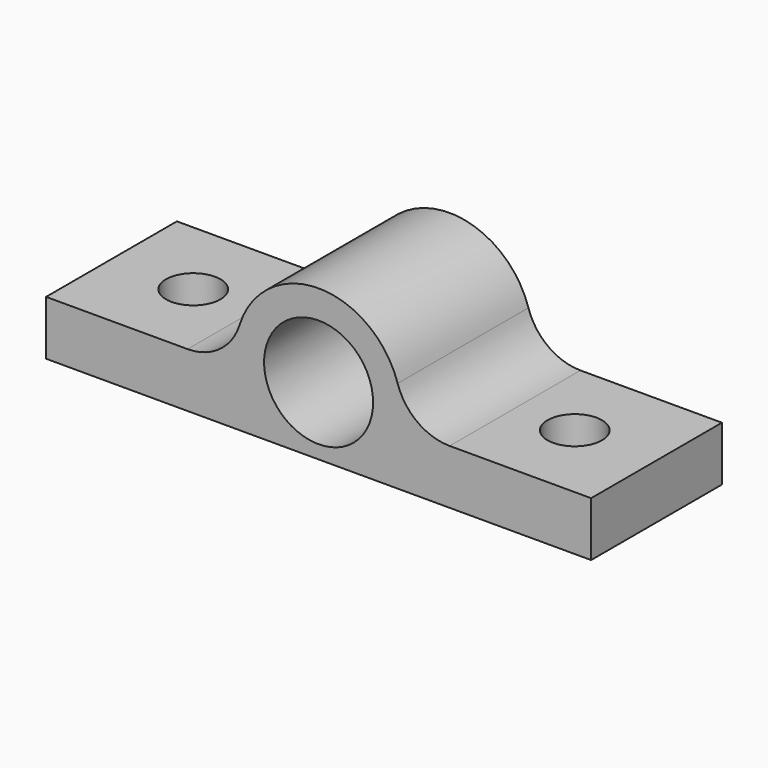
from build123d import *

# Parameters (mm, degrees)
F0_R     = 12.7
F1_DEPTH = 19.05
F2_R     = 12.7
F3_R     = 6.35
F5_DEPTH = 12.7


# Not quite as in the source:
# - the program builds the solid bodies; features that only make, move or delete a surface that nothing else refers to are left out


with BuildPart() as f1:
    # F0 (on Front) → F1 (new body, symmetric)
    with BuildSketch(Plane.XZ):
        with BuildLine():
            Line((-63.5, 12.7), (-63.5, 0))
            Line((-63.5, 0), (63.5, 0))
            Line((63.5, 0), (63.5, 12.7))
            Line((63.5, 12.7), (19.05, 12.7))
            ThreePointArc((19.05, 12.7), (0, 35.1124285501), (-19.05, 12.7))
            Line((-19.05, 12.7), (-63.5, 12.7))
        make_face()
        with Locations((0, 15.8102040816)):
            Circle(F0_R, mode=Mode.SUBTRACT)
    extrude(amount=F1_DEPTH, both=True)

    # F2
    f2_edges = [f1.edges().sort_by_distance(p)[0] for p in [
        (-19.05, 0, 12.7),
        (19.05, 0, 12.7),
    ]]
    fillet(f2_edges, radius=F2_R)

    # F3 (on face) → F5 (cut, through all)
    with BuildSketch(Plane(origin=(0, 0, 0), x_dir=(1, 0, 0), z_dir=(0, 0, -1))):
        with Locations((-44.45, 0)):
            Circle(F3_R)
        with Locations((44.45, 0)):
            Circle(F3_R)
    extrude(amount=-F5_DEPTH, mode=Mode.SUBTRACT)


solid = f1.part
